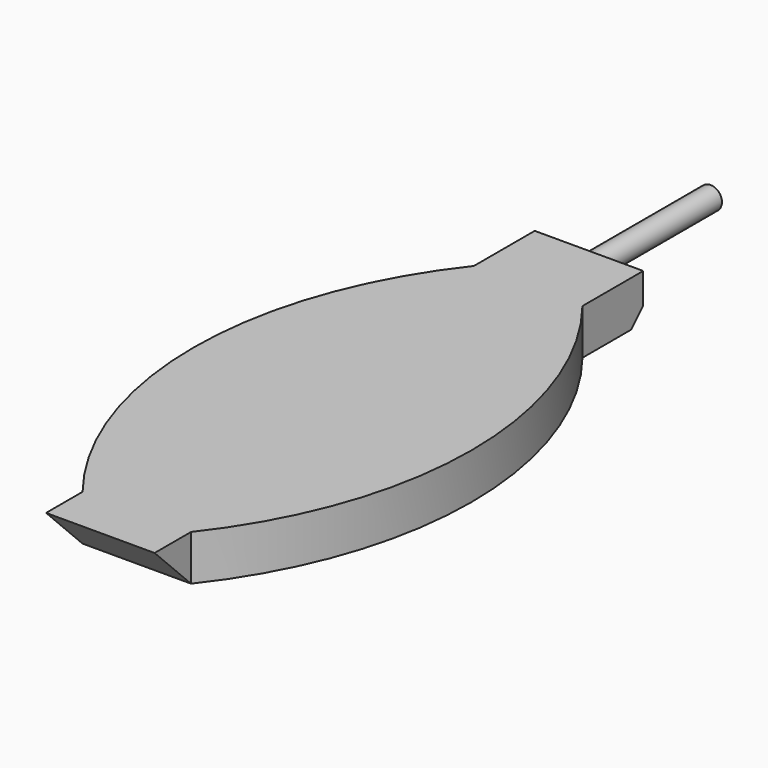
from build123d import *

# Parameters (mm, degrees)
F1_DEPTH    = 3.81
F2_W        = 9.0688861602
F2_H        = 3.81
F3_DEPTH    = 6.35
F4_SIZE     = 1.27
F5_W        = 9.0688861602
F5_H        = 3.81
F6_DEPTH    = 5.08
F7_T1_DEPTH = 35.1971853179
F8_R        = 0.9525
F9_DEPTH    = 12.7


# Not quite as in the source:
# - a fillet or chamfer that OpenCascade refuses, or shapes differently, is made with other operations: its cross-section is extruded or revolved along the edge and cut away or added


with BuildPart() as f1:
    # F0 (on Top) → F1 (new body)
    with BuildSketch(Plane.XY):
        with BuildLine():
            Line((4.5344430801, -2.4189800566), (-4.5344430801, -2.4189800566))
            ThreePointArc((-4.5344430801, -2.4189800566), (-11.6244136954, -22.8629027748), (-4.5344430801, -43.306825493))
            Line((-4.5344430801, -43.306825493), (4.5344430801, -43.306825493))
            ThreePointArc((4.5344430801, -43.306825493), (11.6244136954, -22.8629027748), (4.5344430801, -2.4189800566))
        make_face()
    extrude(amount=F1_DEPTH)

    # F2 (on face) → F3 (join)
    with BuildSketch(Plane(origin=(0, -2.4189800566, 0), x_dir=(-1, 0, 0), z_dir=(0, 1, 0))):
        with Locations((0, 1.905)):
            Rectangle(F2_W, F2_H)
    extrude(amount=F3_DEPTH)

    # F4
    f4_edges = [f1.edges().sort_by_distance(p)[0] for p in [
        (0, 3.93102, 0),
    ]]
    chamfer(f4_edges, length=F4_SIZE)

    # F5 (on face) → F6 (join)
    with BuildSketch(Plane.XZ.offset(43.306825493)):
        with Locations((0, 1.905)):
            Rectangle(F5_W, F5_H)
    extrude(amount=F6_DEPTH)

    # F7: chamfer of 5.08 on 1 edges, made by hand

    # F7_s2 → F7_t1 (cut)
    with BuildSketch(Plane.YZ.offset(-17.598592659)):
        Polygon((-43.306825493, 0), (-48.386825493, 5.08), (-48.386825493, 0), align=None)
    extrude(amount=F7_T1_DEPTH, mode=Mode.SUBTRACT)

    # F8 (on face) → F9 (join)
    with BuildSketch(Plane(origin=(0, 3.9310199434, 0), x_dir=(-1, 0, 0), z_dir=(0, 1, 0))):
        with Locations((0, 2.5457337033)):
            Circle(F8_R)
    extrude(amount=F9_DEPTH)


solid = f1.part
